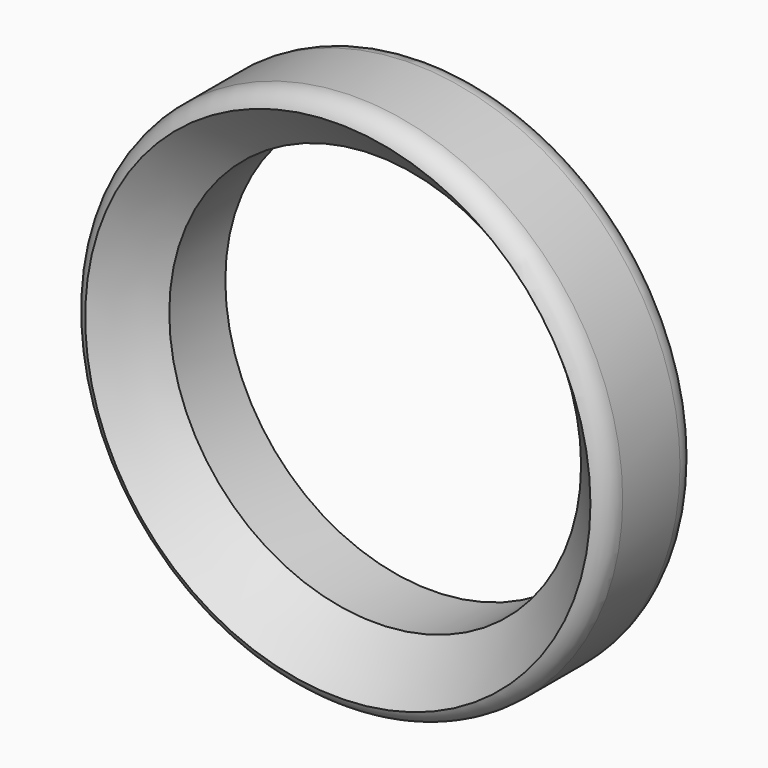
from build123d import *

# Parameters (mm, degrees)
F0_R     = 58.1684180137
F0_R_2   = 44.7813841063
F1_DEPTH = 25.4
F2_SIZE  = 10.16


# Not quite as in the source:
# - a fillet or chamfer that OpenCascade refuses, or shapes differently, is made with other operations: its cross-section is extruded or revolved along the edge and cut away or added


with BuildPart() as f1:
    # F0 (on Front) → F1 (new body)
    with BuildSketch(Plane.XZ):
        Circle(F0_R)
        Circle(F0_R_2, mode=Mode.SUBTRACT)
    extrude(amount=F1_DEPTH)

    # F2
    f2_edges = [f1.edges().sort_by_distance(p)[0] for p in [
        (-44.781384, -25.4, 0),
    ]]
    chamfer(f2_edges, length=F2_SIZE)

    # F3: fillet of radius 5.08 on 2 edges, made by hand

    # F3_s1 → F3_t2 (revolve, cut)
    with BuildSketch(Plane.XY):
        with BuildLine():
            ThreePointArc((54.9413841063, -25.4), (57.2848133567, -23.5329802725), (58.1684180137, -20.669998239))
            Line((58.1684180137, -20.669998239), (58.1684180137, -25.4))
            Line((58.1684180137, -25.4), (54.9413841063, -25.4))
        make_face()
    revolve(axis=Axis((0, -25.4, 0), (0, -1, 0)), mode=Mode.SUBTRACT)

    # F3_s3 → F3_t4 (revolve, cut)
    with BuildSketch(Plane.XY):
        with BuildLine():
            ThreePointArc((53.0884180137, 0), (56.6805204621, -1.4878975516), (58.1684180137, -5.08))
            Line((58.1684180137, -5.08), (58.1684180137, 0))
            Line((58.1684180137, 0), (53.0884180137, 0))
        make_face()
    revolve(axis=Axis((0, 0, 0), (0, -1, 0)), mode=Mode.SUBTRACT)


solid = f1.part
